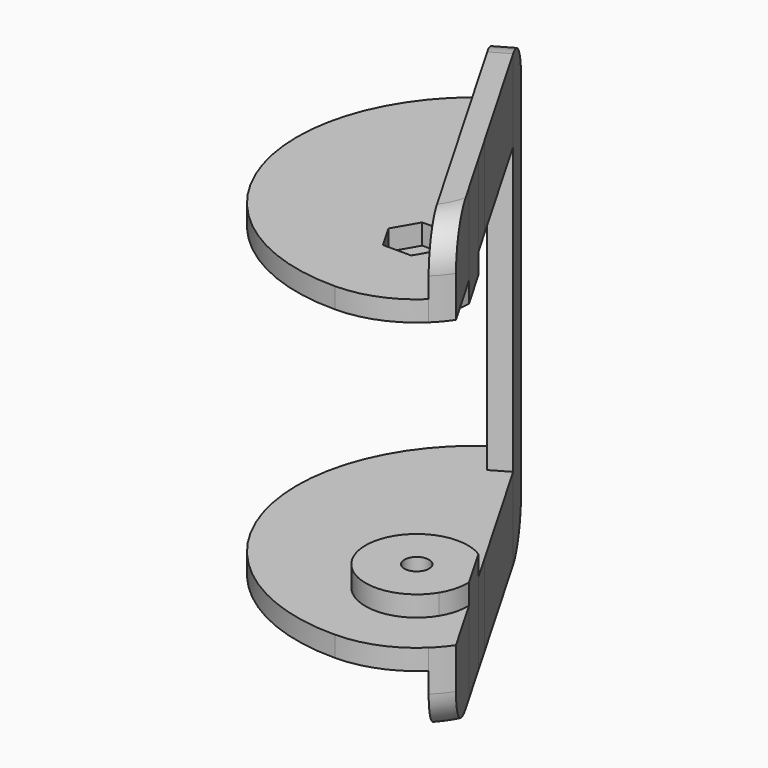
from build123d import *

# Parameters (mm, degrees)
F0_R     = 1.905
F1_DEPTH = 3.175
F2_DEPTH = 3.175
F3_DEPTH = 12.7
F5_DEPTH = 9.525
F6_R     = 6.35
F9_DEPTH = 44.45


with BuildPart() as f1:
    # F0 (on Top) → F1 (new body)
    with BuildSketch(Plane.XY):
        with BuildLine():
            Line((2.1997045256, 3.81), (-0.1821025232, 7.9354108224))
            ThreePointArc((-0.1821025232, 7.9354108224), (-6.8740766425, -3.96875), (6.7812161001, -4.1254108224))
            Line((6.7812161001, -4.1254108224), (4.3994090512, 0))
            Line((4.3994090512, 0), (2.1997045256, -3.81))
            Line((2.1997045256, -3.81), (-2.1997045256, -3.81))
            Line((-2.1997045256, -3.81), (-4.3994090512, 0))
            Line((-4.3994090512, 0), (-2.1997045256, 3.81))
            Line((-2.1997045256, 3.81), (2.1997045256, 3.81))
        make_face()
        with BuildLine():
            ThreePointArc((4.1641356391, 6.7575055034), (2.0762977072, 7.6611287733), (-0.1821025232, 7.9354108224))
            Line((-0.1821025232, 7.9354108224), (2.1997045256, 3.81))
            Line((2.1997045256, 3.81), (4.3994090512, 0))
            Line((4.3994090512, 0), (6.7812161001, -4.1254108224))
            ThreePointArc((6.7812161001, -4.1254108224), (7.672880993, -2.0324378264), (7.9342392518, 0.2274944966))
            Line((7.9342392518, 0.2274944966), (4.1641356391, 6.7575055034))
        make_face()
        Polygon((4.3994090512, 0), (2.1997045256, 3.81), (-2.1997045256, 3.81), (-4.3994090512, 0), (-2.1997045256, -3.81), (2.1997045256, -3.81), align=None)
        Circle(F0_R, mode=Mode.SUBTRACT)
    extrude(amount=-F1_DEPTH)

    # F0 (on Top) → F2 (join)
    with BuildSketch(Plane.XY):
        with BuildLine():
            Line((-1.0837612628, 9.4971295705), (-4.4059530098, 15.2513344687))
            ThreePointArc((-4.4059530098, 15.2513344687), (-15.7183103368, -2.2249371126), (0, -15.875))
            ThreePointArc((0, -15.875), (5.9323031071, -14.7249246125), (11.0050665866, -11.4413344687))
            Line((11.0050665866, -11.4413344687), (6.7812161001, -4.1254108224))
            ThreePointArc((6.7812161001, -4.1254108224), (-6.8740766425, -3.96875), (-0.1821025232, 7.9354108224))
            Line((-0.1821025232, 7.9354108224), (-1.0837612628, 9.4971295705))
        make_face()
        Polygon((-12.5754425904, 29.4013054943), (-4.4059530098, 15.2513344687), (-1.0837612628, 9.4971295705), (1.6658693942, 11.0846295705), (-9.8258119334, 30.9888054943), align=None)
        with BuildLine():
            ThreePointArc((0, -15.875), (-15.7183103368, -2.2249371126), (-4.4059530098, 15.2513344687))
            Line((-4.4059530098, 15.2513344687), (-12.5754425904, 29.4013054943))
            Line((-12.5754425904, 29.4013054943), (-15.7504425904, 34.9005668084))
            ThreePointArc((-15.7504425904, 34.9005668084), (-26.8159478457, 3.6374215932), (0, -15.875))
        make_face()
        with BuildLine():
            Line((1.6658693942, 11.0846295705), (-1.0837612628, 9.4971295705))
            Line((-1.0837612628, 9.4971295705), (-0.1821025232, 7.9354108224))
            ThreePointArc((-0.1821025232, 7.9354108224), (2.0762977072, 7.6611287733), (4.1641356391, 6.7575055034))
            Line((4.1641356391, 6.7575055034), (1.6658693942, 11.0846295705))
        make_face()
        Polygon((-15.7504425904, 34.9005668084), (-12.5754425904, 29.4013054943), (-9.8258119334, 30.9888054943), (-13.0008119334, 36.4880668084), align=None)
        with BuildLine():
            Line((6.7812161001, -4.1254108224), (11.0050665866, -11.4413344687))
            ThreePointArc((11.0050665866, -11.4413344687), (12.1601025371, -10.2052697803), (13.1770447672, -8.8533110305))
            Line((13.1770447672, -8.8533110305), (7.9342392518, 0.2274944966))
            ThreePointArc((7.9342392518, 0.2274944966), (7.672880993, -2.0324378264), (6.7812161001, -4.1254108224))
        make_face()
        with BuildLine():
            ThreePointArc((4.1641356391, 6.7575055034), (2.0762977072, 7.6611287733), (-0.1821025232, 7.9354108224))
            Line((-0.1821025232, 7.9354108224), (2.1997045256, 3.81))
            Line((2.1997045256, 3.81), (4.3994090512, 0))
            Line((4.3994090512, 0), (6.7812161001, -4.1254108224))
            ThreePointArc((6.7812161001, -4.1254108224), (7.672880993, -2.0324378264), (7.9342392518, 0.2274944966))
            Line((7.9342392518, 0.2274944966), (4.1641356391, 6.7575055034))
        make_face()
        with BuildLine():
            Line((2.1997045256, 3.81), (-0.1821025232, 7.9354108224))
            ThreePointArc((-0.1821025232, 7.9354108224), (-6.8740766425, -3.96875), (6.7812161001, -4.1254108224))
            Line((6.7812161001, -4.1254108224), (4.3994090512, 0))
            Line((4.3994090512, 0), (2.1997045256, -3.81))
            Line((2.1997045256, -3.81), (-2.1997045256, -3.81))
            Line((-2.1997045256, -3.81), (-4.3994090512, 0))
            Line((-4.3994090512, 0), (-2.1997045256, 3.81))
            Line((-2.1997045256, 3.81), (2.1997045256, 3.81))
        make_face()
    extrude(amount=F2_DEPTH)

    # F0 (on Top) → F3 (join)
    with BuildSketch(Plane.XY):
        with BuildLine():
            Line((6.7812161001, -4.1254108224), (11.0050665866, -11.4413344687))
            ThreePointArc((11.0050665866, -11.4413344687), (12.1601025371, -10.2052697803), (13.1770447672, -8.8533110305))
            Line((13.1770447672, -8.8533110305), (7.9342392518, 0.2274944966))
            ThreePointArc((7.9342392518, 0.2274944966), (7.672880993, -2.0324378264), (6.7812161001, -4.1254108224))
        make_face()
        with BuildLine():
            Line((1.6658693942, 11.0846295705), (-1.0837612628, 9.4971295705))
            Line((-1.0837612628, 9.4971295705), (-0.1821025232, 7.9354108224))
            ThreePointArc((-0.1821025232, 7.9354108224), (2.0762977072, 7.6611287733), (4.1641356391, 6.7575055034))
            Line((4.1641356391, 6.7575055034), (1.6658693942, 11.0846295705))
        make_face()
        Polygon((-12.5754425904, 29.4013054943), (-4.4059530098, 15.2513344687), (-1.0837612628, 9.4971295705), (1.6658693942, 11.0846295705), (-9.8258119334, 30.9888054943), align=None)
        Polygon((-15.7504425904, 34.9005668084), (-12.5754425904, 29.4013054943), (-9.8258119334, 30.9888054943), (-13.0008119334, 36.4880668084), align=None)
    extrude(amount=F3_DEPTH)

    # F4 (on face) → F5 (join)
    with BuildSketch(Plane.XY.offset(3.175)):
        with BuildLine():
            Line((4.3994090512, 0), (6.7812161001, -4.1254108224))
            ThreePointArc((6.7812161001, -4.1254108224), (7.672880993, -2.0324378264), (7.9342392518, 0.2274944966))
            Line((7.9342392518, 0.2274944966), (4.1641356391, 6.7575055034))
            ThreePointArc((4.1641356391, 6.7575055034), (2.0762977072, 7.6611287733), (-0.1821025232, 7.9354108224))
            Line((-0.1821025232, 7.9354108224), (2.1997045256, 3.81))
            Line((2.1997045256, 3.81), (4.3994090512, 0))
        make_face()
    extrude(amount=F5_DEPTH)

    # F6
    f6_edges = [f1.edges().sort_by_distance(p)[0] for p in [
        (-14.375627, 35.694317, 12.7),
        (12.160103, -10.20527, 12.7),
    ]]
    fillet(f6_edges, radius=F6_R)


with BuildPart() as f8_1:
    # F8: instance of F1
    add(f1.part.mirror(Plane(origin=(-0.1702882742, -0.0983159809, -22.225), x_dir=(1, 0, 0), z_dir=(0, 0, -1))))


with BuildPart() as f1_1:
    add(f1.part)

    add(f8_1.part)  # F9 merges F8_1
    # F0 (on Top) → F9 (join, through all)
    with BuildSketch(Plane.XY):
        Polygon((-15.7504425904, 34.9005668084), (-12.5754425904, 29.4013054943), (-9.8258119334, 30.9888054943), (-13.0008119334, 36.4880668084), align=None)
    extrude(amount=-F9_DEPTH)


solid = f1_1.part
